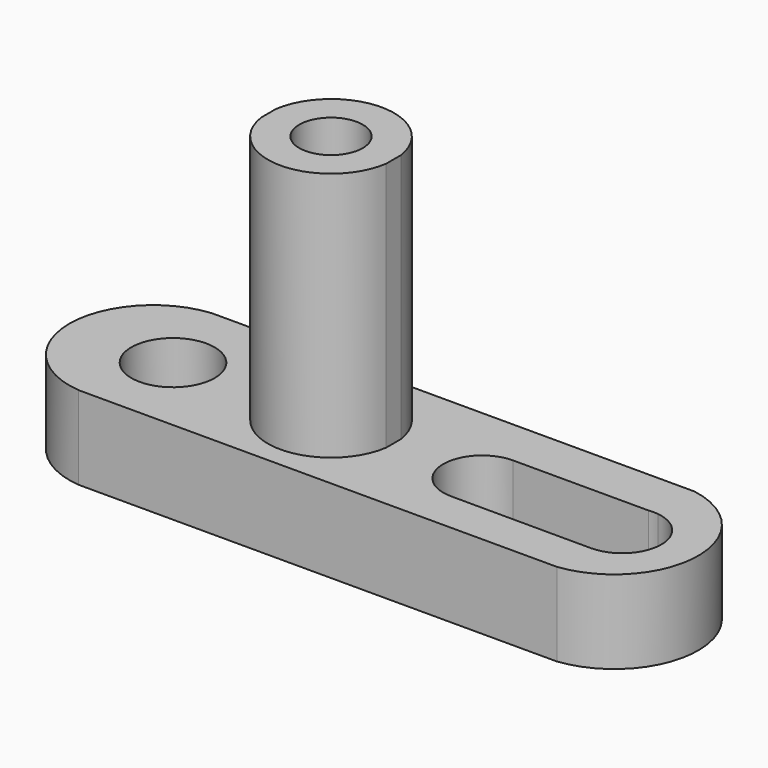
from build123d import *

# Parameters (mm, degrees)
F1_DEPTH  = 25.4
F2_R      = 4.8404450777
F3_DEPTH  = 50.8
F5_DEPTH  = 25.4
F6_DEPTH  = 25.4
F7_R      = 6.3507472709
F8_DEPTH  = 25.4
F10_DEPTH = 38.1
F11_DEPTH = 25.4
F12_DEPTH = 25.4


# Not quite as in the source:
# - a feature names something its author has since deleted; it is built from what else it names


with BuildPart() as f1:
    # F0 (on Front) → F1 (new body)
    with BuildSketch(Plane.XZ):
        Polygon((-101.6, 0), (0, 0), (0, 12.7), (-49.7758105871, 12.7), (-49.7758105871, 50.8), (-68.8258105871, 50.8), (-68.8258105871, 12.7), (-101.6, 12.7), align=None)
    extrude(amount=F1_DEPTH)

    # F2 (on face) → F3 (cut)
    with BuildSketch(Plane.XY.offset(50.8)):
        with Locations((-59.3008105871, -12.7)):
            Circle(F2_R)
    extrude(amount=-F3_DEPTH, mode=Mode.SUBTRACT)

    # F4 (on face) → F5 (cut)
    with BuildSketch(Plane.XY.offset(12.7)):
        with BuildLine():
            ThreePointArc((-35.9137319028, -19.0677542063), (-31.7323936508, -17.3357871934), (-30.0004266379, -13.1544489413))
            ThreePointArc((-30.0004266379, -13.1544489413), (-31.7323936508, -8.9731106893), (-35.9137319028, -7.2411436764))
            ThreePointArc((-35.9137319028, -7.2411436764), (-41.8270371678, -13.1544489413), (-35.9137319028, -19.0677542063))
        make_face()
        with BuildLine():
            ThreePointArc((-35.9137319028, -7.2411436764), (-31.7323936508, -8.9731106893), (-30.0004266379, -13.1544489413))
            ThreePointArc((-30.0004266379, -13.1544489413), (-31.7323936508, -17.3357871934), (-35.9137319028, -19.0677542063))
            Line((-35.9137319028, -19.0677542063), (-14.5683543234, -19.1081041901))
            ThreePointArc((-14.5683543234, -19.1081041901), (-20.5006521622, -13.5013264467), (-15.2608531919, -7.2425229617))
            Line((-15.2608531919, -7.2425229617), (-35.9137319028, -7.2411436632))
        make_face()
        with BuildLine():
            Line((-13.852556963, -7.2426170145), (-15.2608531919, -7.2425229617))
            ThreePointArc((-15.2608531919, -7.2425229617), (-20.5006521622, -13.5013264467), (-14.5683543234, -19.1081041901))
            ThreePointArc((-14.5683543234, -19.1081041901), (-10.3512033015, -17.3683036228), (-8.603434015, -13.1544489413))
            ThreePointArc((-8.603434015, -13.1544489413), (-10.1050918857, -9.2015054667), (-13.852556963, -7.2426170145))
        make_face()
        with BuildLine():
            ThreePointArc((-13.852556963, -7.2426170145), (-14.5567022867, -7.2007830685), (-15.2608531919, -7.2425229617))
            Line((-15.2608531919, -7.2425229617), (-13.852556963, -7.2426170145))
        make_face()
        with BuildLine():
            ThreePointArc((-14.0938774664, 0), (-3.3585658021, -12.9691778388), (-14.712910818, -25.4))
            Line((-14.712910818, -25.4), (0, -25.4))
            Line((0, -25.4), (0, 0))
            Line((0, 0), (-14.0938774664, 0))
        make_face()
    extrude(amount=-F5_DEPTH, mode=Mode.SUBTRACT)

    # F4 (on face) → F6 (cut)
    with BuildSketch(Plane.XY.offset(12.7)):
        with BuildLine():
            ThreePointArc((-35.9137319028, -19.0677542063), (-31.7323936508, -17.3357871934), (-30.0004266379, -13.1544489413))
            ThreePointArc((-30.0004266379, -13.1544489413), (-31.7323936508, -8.9731106893), (-35.9137319028, -7.2411436764))
            ThreePointArc((-35.9137319028, -7.2411436764), (-41.8270371678, -13.1544489413), (-35.9137319028, -19.0677542063))
        make_face()
        with BuildLine():
            ThreePointArc((-35.9137319028, -7.2411436764), (-31.7323936508, -8.9731106893), (-30.0004266379, -13.1544489413))
            ThreePointArc((-30.0004266379, -13.1544489413), (-31.7323936508, -17.3357871934), (-35.9137319028, -19.0677542063))
            Line((-35.9137319028, -19.0677542063), (-14.5683543234, -19.1081041901))
            ThreePointArc((-14.5683543234, -19.1081041901), (-20.5006521622, -13.5013264467), (-15.2608531919, -7.2425229617))
            Line((-15.2608531919, -7.2425229617), (-35.9137319028, -7.2411436632))
        make_face()
        with BuildLine():
            Line((-13.852556963, -7.2426170145), (-15.2608531919, -7.2425229617))
            ThreePointArc((-15.2608531919, -7.2425229617), (-20.5006521622, -13.5013264467), (-14.5683543234, -19.1081041901))
            ThreePointArc((-14.5683543234, -19.1081041901), (-10.3512033015, -17.3683036228), (-8.603434015, -13.1544489413))
            ThreePointArc((-8.603434015, -13.1544489413), (-10.1050918857, -9.2015054667), (-13.852556963, -7.2426170145))
        make_face()
        with BuildLine():
            ThreePointArc((-13.852556963, -7.2426170145), (-14.5567022867, -7.2007830685), (-15.2608531919, -7.2425229617))
            Line((-15.2608531919, -7.2425229617), (-13.852556963, -7.2426170145))
        make_face()
    extrude(amount=-F6_DEPTH, mode=Mode.SUBTRACT)

    # F7 (on face) → F8 (cut)
    with BuildSketch(Plane.XY.offset(12.7)):
        with Locations((-83.2697451115, -12.8449322656)):
            Circle(F7_R)
        with BuildLine():
            ThreePointArc((-87.6296867998, -25.4), (-99.1786550293, -12.7), (-87.6296867998, 0))
            Line((-87.6296867998, 0), (-101.6, 0))
            Line((-101.6, 0), (-101.6, -25.4))
            Line((-101.6, -25.4), (-87.6296867998, -25.4))
        make_face()
    extrude(amount=-F8_DEPTH, mode=Mode.SUBTRACT)

    # F9 (on face) → F10 (cut)
    with BuildSketch(Plane.XY.offset(50.8)):
        with BuildLine():
            ThreePointArc((-68.8258105871, -11.3028298429), (-59.3008105871, -3.0730737279), (-49.7758105871, -11.3028298429))
            Line((-49.7758105871, -11.3028298429), (-49.7758105871, 0))
            Line((-49.7758105871, 0), (-68.8258105871, 0))
            Line((-68.8258105871, 0), (-68.8258105871, -11.3028298429))
        make_face()
        with BuildLine():
            Line((-49.7758105871, -25.4), (-49.7758105871, -14.0971701571))
            ThreePointArc((-49.7758105871, -14.0971701571), (-59.3008105871, -22.3269262721), (-68.8258105871, -14.0971701571))
            Line((-68.8258105871, -14.0971701571), (-68.8258105871, -25.4))
            Line((-68.8258105871, -25.4), (-49.7758105871, -25.4))
        make_face()
    extrude(amount=-F10_DEPTH, mode=Mode.SUBTRACT)


with BuildPart() as f11:
    # F7 (on face) → F11 (new body)
    with BuildSketch(Plane.XY.offset(12.7)):
        with Locations((-83.2697451115, -12.8449322656)):
            Circle(F7_R)
    extrude(amount=F11_DEPTH)

    # F12 (cut): a face of the model
    f12_faces = [f11.faces().sort_by_distance(p)[0] for p in [
        (-83.2697451115, -12.8449322656, 38.1),
    ]]
    extrude(f12_faces, amount=-F12_DEPTH, mode=Mode.SUBTRACT)


solid = f1.part
